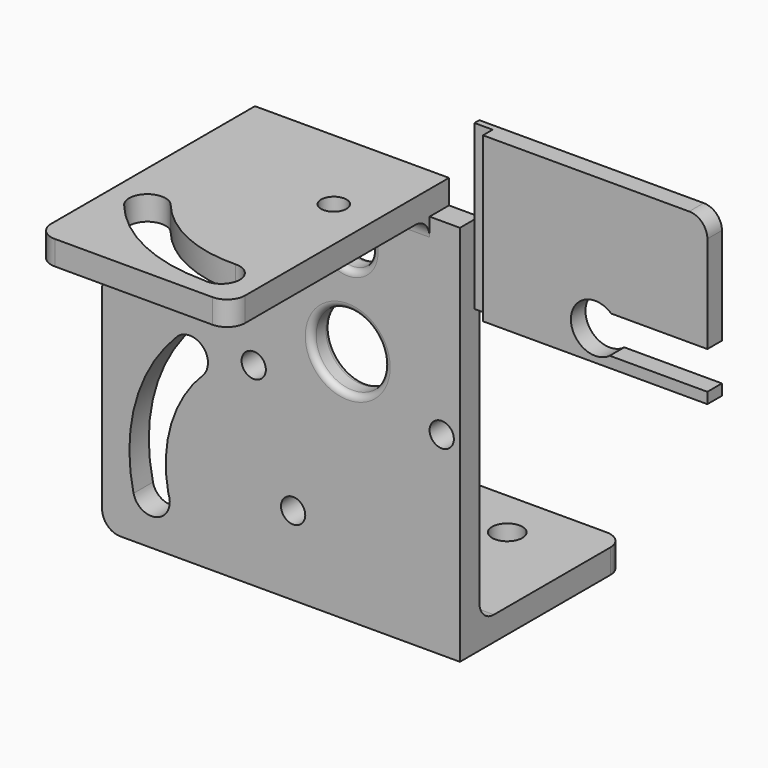
from build123d import *

# Parameters (mm, degrees)
F0_R      = 2
F0_R_2    = 6
F0_R_3    = 4
F1_DEPTH  = 4
F3_DEPTH  = 45
F4_R      = 4
F5_DEPTH  = 3.001
F6_W      = 18
F6_H      = 6.2
F6_W_2    = 40
F6_H_2    = 18
F7_DEPTH  = 4.001
F8_W      = 37
F8_H      = 4
F9_DEPTH  = 30
F10_R     = 2.5
F11_DEPTH = 4.001
F12_W     = 32
F12_H     = 45
F12_R     = 2.1
F13_DEPTH = 4
F14_R     = 1
F15_R     = 3
F16_R     = 2.99999


# Not quite as in the source:
# - a fillet or chamfer is up to 0.001 mm smaller than in the source, because OpenCascade refuses the exact size


with BuildPart() as f1:
    # F0 (on Front) → F1 (new body)
    with BuildSketch(Plane.XZ):
        Polygon((-40.5, -32), (-18.5, -32), (18.5, -32), (18.5, 0), (18.5, 31), (-18.5, 31), (-18.5, 6), (-40.5, 6), align=None)
        with BuildLine():
            ThreePointArc((-28.1833260933, 0), (-24.0098257239, 0.092032915), (-23.7739154785, -4.0758108617))
            ThreePointArc((-23.7739154785, -4.0758108617), (-29.0960224362, -12.9049296767), (-29.5751173341, -23.2029212089))
            ThreePointArc((-29.5751173341, -23.2029212089), (-31.4417329452, -27.2483725045), (-35.3144480282, -25.0456451244))
            ThreePointArc((-35.3144480282, -25.0456451244), (-34.9679215076, -11.6062828988), (-28.1833260933, 0))
        make_face(mode=Mode.SUBTRACT)
        with Locations((-9, -19)):
            Circle(F0_R, mode=Mode.SUBTRACT)
        with Locations((-15.5, 0)):
            Circle(F0_R, mode=Mode.SUBTRACT)
        with Locations((0, 7)):
            Circle(F0_R_2, mode=Mode.SUBTRACT)
        with Locations((15.5, 0)):
            Circle(F0_R, mode=Mode.SUBTRACT)
        with Locations((0, 23)):
            Circle(F0_R_3, mode=Mode.SUBTRACT)
    extrude(amount=F1_DEPTH)

    # F2 (on Top) → F3 (join)
    with BuildSketch(Plane.XY):
        Polygon((18.5, 0), (18.5, -1), (21.5, -1), (21.5, -3), (58.5, -3), (58.5, 0), align=None)
    extrude(amount=F3_DEPTH)

    # F4 (on face) → F5 (cut, through all)
    with BuildSketch(Plane.XZ.offset(3)):
        with Locations((40, 23)):
            Circle(F4_R)
    extrude(amount=-F5_DEPTH, mode=Mode.SUBTRACT)

    # F6 (on face) → F7 (cut, through all)
    with BuildSketch(Plane.XZ.offset(4)):
        with Locations((-9.5, 23.1)):
            Rectangle(F6_W, F6_H)
        with Locations((49.5, 22.9)):
            Rectangle(F6_W, F6_H)
        with Locations((38.5, 9)):
            Rectangle(F6_W_2, F6_H_2)
    extrude(amount=-F7_DEPTH, mode=Mode.SUBTRACT)

    # F8 (on face) → F9 (join)
    with BuildSketch(Plane(origin=(0, 0, 0), x_dir=(-1, 0, 0), z_dir=(0, 1, 0))):
        with Locations((0, -30)):
            Rectangle(F8_W, F8_H)
    extrude(amount=F9_DEPTH)

    # F10 (on face) → F11 (cut, through all)
    with BuildSketch(Plane.XY.offset(-28)):
        with Locations((5.5, 22)):
            Circle(F10_R)
    extrude(amount=-F11_DEPTH, mode=Mode.SUBTRACT)

    # F12 (on face) → F13 (join)
    with BuildSketch(Plane.XY.offset(31)):
        with Locations((-2.5, -22.5)):
            Rectangle(F12_W, F12_H)
        with BuildLine():
            ThreePointArc((6.6234089411, -41.9997179658), (-5.0413076784, -39.4089782063), (-14.4456133354, -32.0376430883))
            ThreePointArc((-14.4456133354, -32.0376430883), (-13.9930410249, -27.8021990866), (-9.7612789693, -28.2879948179))
            ThreePointArc((-9.7612789693, -28.2879948179), (-2.2263981239, -34.1010464578), (7.1005801395, -35.9914102312))
            ThreePointArc((7.1005801395, -35.9914102312), (10.2089825884, -39.2613770976), (6.6234089411, -41.9997179658))
        make_face(mode=Mode.SUBTRACT)
        with Locations((6.5, -15)):
            Circle(F12_R, mode=Mode.SUBTRACT)
    extrude(amount=F13_DEPTH)

    # F14
    f14_edges = [f1.edges().sort_by_distance(p)[0] for p in [
        (6, -2, 7),
        (-6, 0, 7),
        (-6, -4, 7),
        (3.996861, -4, 22.841575),
        (-2.4, -2, 26.2),
        (3.996861, 0, 22.841575),
        (-2.645751, -2, 20),
        (-10.45, -4, 26.2),
        (-18.5, -2, 26.2),
        (-10.45, 0, 26.2),
        (-10.572876, 0, 20),
    ]]
    fillet(f14_edges, radius=F14_R)

    # F15
    f15_edges = [f1.edges().sort_by_distance(p)[0] for p in [
        (0, 0, -28),
        (-40.5, -2, 6),
        (-40.5, -2, -32),
        (18.5, 30, -30),
        (-18.5, 30, -30),
        (58.5, -1.5, 45),
        (-18.5, -45, 33),
        (13.5, -45, 33),
    ]]
    fillet(f15_edges, radius=F15_R)

    # F16 (radius 3 in the source; OpenCascade refuses exactly that, so slightly less here)
    f16_edges = [f1.edges().sort_by_distance(p)[0] for p in [
        (-2.5, -4, 31),
        (-18.5, -2, 6),
    ]]
    fillet(f16_edges, radius=F16_R)


solid = f1.part
